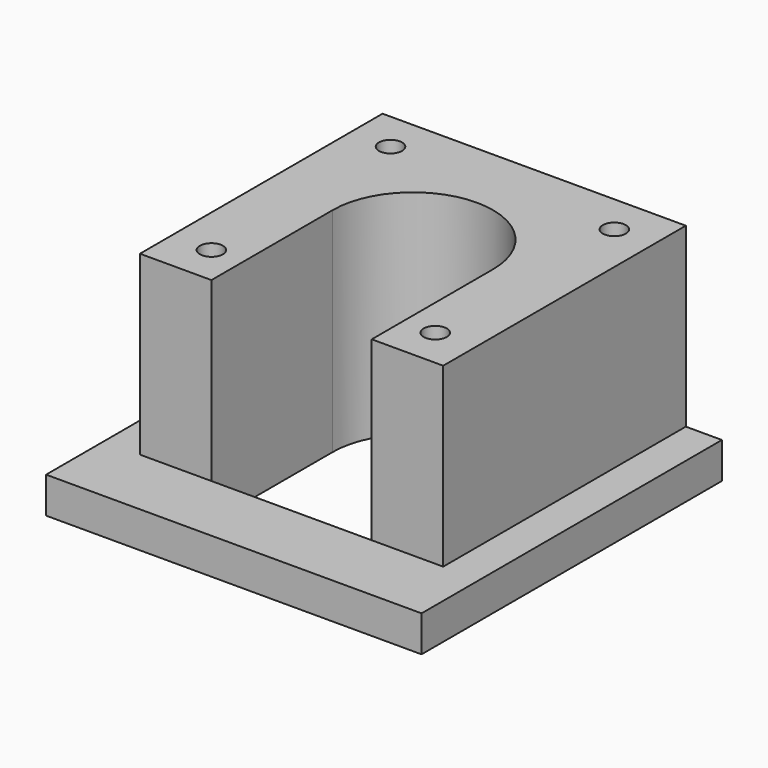
from build123d import *

# Parameters (mm, degrees)
F0_W     = 52
F0_H     = 52
F1_DEPTH = 5
F2_W     = 42
F2_H     = 42
F3_DEPTH = 24.5
F4_R     = 1.6
F5_DEPTH = 29.5


# Not quite as in the source:
# - a feature names something its author has since deleted; it is built from what else it names


with BuildPart() as f1:
    # F0 (on Top) → F1 (new body)
    with BuildSketch(Plane.XY):
        Rectangle(F0_W, F0_H)
    extrude(amount=F1_DEPTH)

    # F2 (on face) → F3 (join)
    with BuildSketch(Plane.XY.offset(5)):
        with Locations((0, 5)):
            Rectangle(F2_W, F2_H)
    extrude(amount=F3_DEPTH)

    # F4 (on face) → F5 (cut, through all)
    with BuildSketch(Plane.XY.offset(29.5)):
        with Locations((-15.5, 20.5)):
            Circle(F4_R)
        with Locations((15.5, 20.5)):
            Circle(F4_R)
        with Locations((-15.5, -10.5)):
            Circle(F4_R)
        with Locations((15.5, -10.5)):
            Circle(F4_R)
        with BuildLine():
            ThreePointArc((-11.1, 5), (0, -6.1), (11.1, 5))
            ThreePointArc((11.1, 5), (0, 16.1), (-11.1, 5))
        make_face()
        with BuildLine():
            Line((11.1, -16), (11.1, 5))
            ThreePointArc((11.1, 5), (0, -6.1), (-11.1, 5))
            Line((-11.1, 5), (-11.1, -16))
            Line((-11.1, -16), (11.1, -16))
        make_face()
    extrude(amount=-F5_DEPTH, mode=Mode.SUBTRACT)


solid = f1.part
